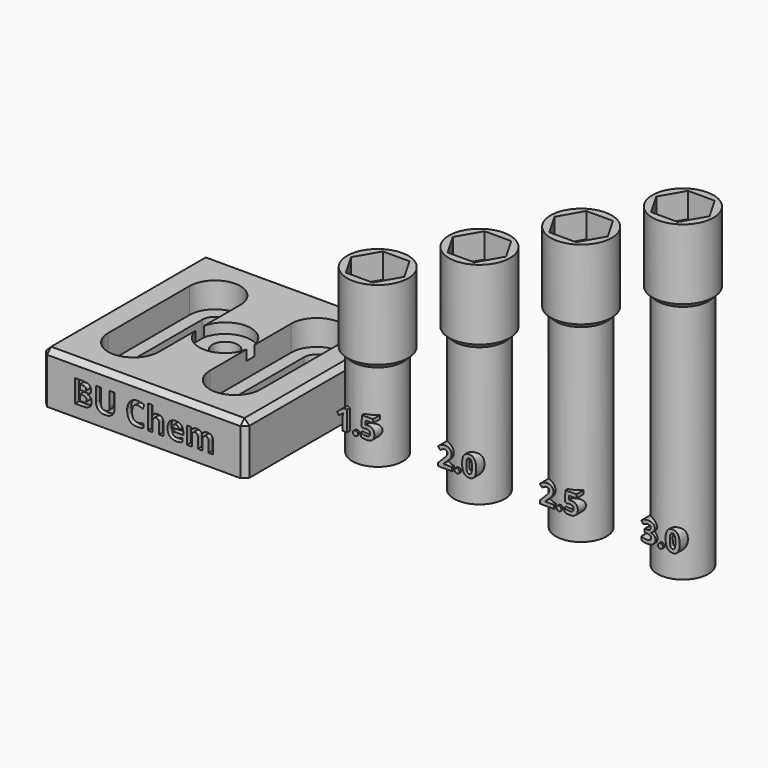
from build123d import *

# Parameters (mm, degrees)
F0_W          = 50.8
F0_H          = 50.8
F0_R          = 3.175
F1_DEPTH      = 12.7
F3_DEPTH      = 6.35
F2_R          = 3.175
F4_DEPTH      = 2.54
F5_SIZE       = 1.27
F6_DEPTH      = 5.08
F7_TEXT_SIZE  = 7.8593141451
F8_DEPTH      = 1.27
F0_R_2        = 6.35
F0_R_3        = 3.429
F9_DEPTH      = 47.244
F10_DEPTH     = 21.844
F11_DEPTH     = 34.544
F12_DEPTH     = 59.944
F13_R         = 7.62
F13_R_2       = 6.35
F13_R_3       = 3.429
F14_DEPTH     = 18.796
F15_R         = 7.62
F15_R_2       = 6.35
F15_R_3       = 3.429
F16_DEPTH     = 18.796
F17_R         = 7.62
F17_R_2       = 6.35
F17_R_3       = 3.429
F18_DEPTH     = 18.796
F19_R         = 7.62
F19_R_2       = 6.35
F19_R_3       = 3.429
F20_DEPTH     = 18.796
F21_SIZE      = 1.26999
F21_2_SIZE    = 1.26999
F21_3_SIZE    = 1.26999
F21_4_SIZE    = 1.26999
F22_R         = 3.429
F23_DEPTH     = 6.223
F24_R         = 3.429
F25_DEPTH     = 6.223
F26_R         = 3.429
F27_DEPTH     = 6.223
F28_R         = 3.429
F29_DEPTH     = 6.223
F31_TEXT_SIZE = 7.0555555556
F32_DEPTH     = 3.175
F33_DEPTH     = 3.175
F34_DEPTH     = 3.175
F35_DEPTH     = 3.175


# Not quite as in the source:
# - a fillet or chamfer is up to 0.001 mm smaller than in the source, because OpenCascade refuses the exact size
# - Text() gives the source's letters only with a copy of the font that has no kerning and outlines rounded to 1/6400 em; it was checked with that copy


with BuildPart() as f1:
    # F0 (on Top) → F1 (new body)
    with BuildSketch(Plane.XY):
        Rectangle(F0_W, F0_H)
        with BuildLine():
            Line((-9.525, 12.7), (-9.525, -12.7))
            ThreePointArc((-9.525, -12.7), (-12.7, -15.875), (-15.875, -12.7))
            Line((-15.875, -12.7), (-15.875, 12.7))
            ThreePointArc((-15.875, 12.7), (-12.7, 15.875), (-9.525, 12.7))
        make_face(mode=Mode.SUBTRACT)
        Polygon((0, 6.604), (5.7192317666, 3.302), (5.7192317666, -3.302), (0, -6.604), (-5.7192317666, -3.302), (-5.7192317666, 3.302), align=None, mode=Mode.SUBTRACT)
        with BuildLine():
            Line((15.875, 12.7), (15.875, -12.7))
            ThreePointArc((15.875, -12.7), (12.7, -15.875), (9.525, -12.7))
            Line((9.525, -12.7), (9.525, 12.7))
            ThreePointArc((9.525, 12.7), (12.7, 15.875), (15.875, 12.7))
        make_face(mode=Mode.SUBTRACT)
        Polygon((5.7192317666, -3.302), (5.7192317666, 3.302), (0, 6.604), (-5.7192317666, 3.302), (-5.7192317666, -3.302), (0, -6.604), align=None)
        Circle(F0_R, mode=Mode.SUBTRACT)
    extrude(amount=F1_DEPTH)

    # F2 (on face) → F3 (cut)
    with BuildSketch(Plane.XY.offset(12.7)):
        with BuildLine():
            ThreePointArc((-9.525, 7.200738686), (-7.200738686, 9.525), (-6.35, 12.7))
            ThreePointArc((-6.35, 12.7), (-12.7, 19.05), (-19.05, 12.7))
            ThreePointArc((-19.05, 12.7), (-18.199261314, 9.525), (-15.875, 7.200738686))
            Line((-15.875, 7.200738686), (-15.875, 12.7))
            ThreePointArc((-15.875, 12.7), (-12.7, 15.875), (-9.525, 12.7))
            Line((-9.525, 12.7), (-9.525, 7.200738686))
        make_face()
        with BuildLine():
            Line((-6.35, 1.2763342039), (-6.35, 12.7))
            ThreePointArc((-6.35, 12.7), (-7.200738686, 9.525), (-9.525, 7.200738686))
            Line((-9.525, 7.200738686), (-9.525, -7.200738686))
            ThreePointArc((-9.525, -7.200738686), (-7.200738686, -9.525), (-6.35, -12.7))
            Line((-6.35, -12.7), (-6.35, -1.2763342039))
            ThreePointArc((-6.35, -1.2763342039), (-6.477, 0), (-6.35, 1.2763342039))
        make_face()
        with BuildLine():
            ThreePointArc((-15.875, 7.200738686), (-18.199261314, 9.525), (-19.05, 12.7))
            Line((-19.05, 12.7), (-19.05, -12.7))
            ThreePointArc((-19.05, -12.7), (-18.199261314, -9.525), (-15.875, -7.200738686))
            Line((-15.875, -7.200738686), (-15.875, 7.200738686))
        make_face()
        with BuildLine():
            ThreePointArc((-15.875, 7.200738686), (-12.7, 6.35), (-9.525, 7.200738686))
            Line((-9.525, 7.200738686), (-9.525, 12.7))
            ThreePointArc((-9.525, 12.7), (-12.7, 15.875), (-15.875, 12.7))
            Line((-15.875, 12.7), (-15.875, 7.200738686))
        make_face()
        with BuildLine():
            Line((-6.35, -1.2763342039), (-6.35, 1.2763342039))
            ThreePointArc((-6.35, 1.2763342039), (-6.477, 0), (-6.35, -1.2763342039))
        make_face()
        with BuildLine():
            ThreePointArc((-15.875, -7.200738686), (-18.199261314, -9.525), (-19.05, -12.7))
            ThreePointArc((-19.05, -12.7), (-12.7, -19.05), (-6.35, -12.7))
            ThreePointArc((-6.35, -12.7), (-7.200738686, -9.525), (-9.525, -7.200738686))
            Line((-9.525, -7.200738686), (-9.525, -12.7))
            ThreePointArc((-9.525, -12.7), (-12.7, -15.875), (-15.875, -12.7))
            Line((-15.875, -12.7), (-15.875, -7.200738686))
        make_face()
        with BuildLine():
            Line((-9.525, -12.7), (-9.525, -7.200738686))
            ThreePointArc((-9.525, -7.200738686), (-12.7, -6.35), (-15.875, -7.200738686))
            Line((-15.875, -7.200738686), (-15.875, -12.7))
            ThreePointArc((-15.875, -12.7), (-12.7, -15.875), (-9.525, -12.7))
        make_face()
        with BuildLine():
            Line((6.35, 12.7), (6.35, 1.2763342039))
            ThreePointArc((6.35, 1.2763342039), (6.4451717976, 0.6413185636), (6.477, 0))
            ThreePointArc((6.477, 0), (6.4451717976, -0.6413185636), (6.35, -1.2763342039))
            Line((6.35, -1.2763342039), (6.35, -12.7))
            ThreePointArc((6.35, -12.7), (7.200738686, -9.525), (9.525, -7.200738686))
            Line((9.525, -7.200738686), (9.525, 7.200738686))
            ThreePointArc((9.525, 7.200738686), (7.200738686, 9.525), (6.35, 12.7))
        make_face()
        with BuildLine():
            ThreePointArc((6.477, 0), (6.4451717976, 0.6413185636), (6.35, 1.2763342039))
            Line((6.35, 1.2763342039), (6.35, -1.2763342039))
            ThreePointArc((6.35, -1.2763342039), (6.4451717976, -0.6413185636), (6.477, 0))
        make_face()
        with BuildLine():
            ThreePointArc((19.05, 12.7), (12.7, 19.05), (6.35, 12.7))
            ThreePointArc((6.35, 12.7), (7.200738686, 9.525), (9.525, 7.200738686))
            Line((9.525, 7.200738686), (9.525, 12.7))
            ThreePointArc((9.525, 12.7), (12.7, 15.875), (15.875, 12.7))
            Line((15.875, 12.7), (15.875, 7.200738686))
            ThreePointArc((15.875, 7.200738686), (18.199261314, 9.525), (19.05, 12.7))
        make_face()
        with BuildLine():
            Line((19.05, -12.7), (19.05, 12.7))
            ThreePointArc((19.05, 12.7), (18.199261314, 9.525), (15.875, 7.200738686))
            Line((15.875, 7.200738686), (15.875, -7.200738686))
            ThreePointArc((15.875, -7.200738686), (18.199261314, -9.525), (19.05, -12.7))
        make_face()
        with BuildLine():
            Line((9.525, 12.7), (9.525, 7.200738686))
            ThreePointArc((9.525, 7.200738686), (12.7, 6.35), (15.875, 7.200738686))
            Line((15.875, 7.200738686), (15.875, 12.7))
            ThreePointArc((15.875, 12.7), (12.7, 15.875), (9.525, 12.7))
        make_face()
        with BuildLine():
            ThreePointArc((9.525, -7.200738686), (7.200738686, -9.525), (6.35, -12.7))
            ThreePointArc((6.35, -12.7), (12.7, -19.05), (19.05, -12.7))
            ThreePointArc((19.05, -12.7), (18.199261314, -9.525), (15.875, -7.200738686))
            Line((15.875, -7.200738686), (15.875, -12.7))
            ThreePointArc((15.875, -12.7), (12.7, -15.875), (9.525, -12.7))
            Line((9.525, -12.7), (9.525, -7.200738686))
        make_face()
        with BuildLine():
            ThreePointArc((15.875, -7.200738686), (12.7, -6.35), (9.525, -7.200738686))
            Line((9.525, -7.200738686), (9.525, -12.7))
            ThreePointArc((9.525, -12.7), (12.7, -15.875), (15.875, -12.7))
            Line((15.875, -12.7), (15.875, -7.200738686))
        make_face()
    extrude(amount=-F3_DEPTH, mode=Mode.SUBTRACT)

    # F2 (on face) → F4 (cut)
    with BuildSketch(Plane.XY.offset(12.7)):
        with BuildLine():
            Line((-6.35, -1.2763342039), (-6.35, 1.2763342039))
            ThreePointArc((-6.35, 1.2763342039), (-6.477, 0), (-6.35, -1.2763342039))
        make_face()
        with BuildLine():
            ThreePointArc((6.35, 1.2763342039), (0, 6.477), (-6.35, 1.2763342039))
            Line((-6.35, 1.2763342039), (-6.35, -1.2763342039))
            ThreePointArc((-6.35, -1.2763342039), (0, -6.477), (6.35, -1.2763342039))
            Line((6.35, -1.2763342039), (6.35, 1.2763342039))
        make_face()
        Circle(F2_R, mode=Mode.SUBTRACT)
        with BuildLine():
            ThreePointArc((6.477, 0), (6.4451717976, 0.6413185636), (6.35, 1.2763342039))
            Line((6.35, 1.2763342039), (6.35, -1.2763342039))
            ThreePointArc((6.35, -1.2763342039), (6.4451717976, -0.6413185636), (6.477, 0))
        make_face()
    extrude(amount=-F4_DEPTH, mode=Mode.SUBTRACT)

    # F5
    f5_edges = [f1.edges().sort_by_distance(p)[0] for p in [
        (0, -25.4, 12.7),
        (-25.4, 0, 12.7),
        (0, 25.4, 12.7),
        (25.4, 0, 12.7),
        (-25.4, -25.4, 6.35),
        (25.4, -25.4, 6.35),
        (-25.4, 25.4, 6.35),
        (25.4, 25.4, 6.35),
    ]]
    chamfer(f5_edges, length=F5_SIZE)

    # F0 (on Top) → F6 (cut)
    with BuildSketch(Plane.XY):
        Polygon((5.7192317666, -3.302), (5.7192317666, 3.302), (0, 6.604), (-5.7192317666, 3.302), (-5.7192317666, -3.302), (0, -6.604), align=None)
        Circle(F0_R, mode=Mode.SUBTRACT)
    extrude(amount=F6_DEPTH, mode=Mode.SUBTRACT)

    # F7 (on face) → F8 (cut)
    with BuildSketch(Plane.XZ.offset(25.4)):
        with Locations((-17.8596773858, 2.9821679927)):
            Text('BU Chem', F7_TEXT_SIZE, font='Open Sans', font_style=FontStyle.BOLD, text_align=(TextAlign.LEFT, TextAlign.BOTTOM))
    extrude(amount=-F8_DEPTH, mode=Mode.SUBTRACT)


with BuildPart() as f9:
    # F0 (on Top) → F9 (new body)
    with BuildSketch(Plane.XY):
        with Locations((88.9, 0)):
            Circle(F0_R_2)
        with Locations((88.9, 0)):
            Circle(F0_R_3, mode=Mode.SUBTRACT)
    extrude(amount=F9_DEPTH)

    # F17 (on face) → F18 (join)
    with BuildSketch(Plane.XY.offset(47.244)):
        with Locations((88.9, 0)):
            Circle(F17_R)
        with Locations((88.9, 0)):
            Circle(F17_R_2, mode=Mode.SUBTRACT)
        with Locations((88.9, 0)):
            Circle(F17_R_2)
        with Locations((88.9, 0)):
            Circle(F17_R_3, mode=Mode.SUBTRACT)
    extrude(amount=F18_DEPTH)

    # F21 (size 1.27 in the source; OpenCascade refuses exactly that, so slightly less here)
    f21_edges = [f9.edges().sort_by_distance(p)[0] for p in [
        (81.28, 0, 47.244),
    ]]
    chamfer(f21_edges, length=F21_SIZE)

    # F26 (on face) → F27 (cut)
    with BuildSketch(Plane.XY.offset(66.04)):
        Polygon((92.2274, -5.7632258571), (95.5548, 0), (92.2274, 5.7632258571), (85.5726, 5.7632258571), (82.2452, 0), (85.5726, -5.7632258571), align=None)
        with Locations((88.9, 0)):
            Circle(F26_R, mode=Mode.SUBTRACT)
    extrude(amount=-F27_DEPTH, mode=Mode.SUBTRACT)

    # F31 (on offset) → F34 (join)
    with BuildSketch(Plane.XZ.offset(6.858)):
        with Locations((83.7962977431, 6.35)):
            Text('2.5', F31_TEXT_SIZE, font='Open Sans', font_style=FontStyle.BOLD, text_align=(TextAlign.LEFT, TextAlign.BOTTOM))
    extrude(amount=-F34_DEPTH)


with BuildPart() as f10:
    # F0 (on Top) → F10 (new body)
    with BuildSketch(Plane.XY):
        with Locations((38.1, 0)):
            Circle(F0_R_2)
        with Locations((38.1, 0)):
            Circle(F0_R_3, mode=Mode.SUBTRACT)
    extrude(amount=F10_DEPTH)

    # F13 (on face) → F14 (join)
    with BuildSketch(Plane.XY.offset(21.844)):
        with Locations((38.1, 0)):
            Circle(F13_R)
        with Locations((38.1, 0)):
            Circle(F13_R_2, mode=Mode.SUBTRACT)
        with Locations((38.1, 0)):
            Circle(F13_R_2)
        with Locations((38.1, 0)):
            Circle(F13_R_3, mode=Mode.SUBTRACT)
    extrude(amount=F14_DEPTH)

    # F21#2 (size 1.27 in the source; OpenCascade refuses exactly that, so slightly less here)
    f21_2_edges = [f10.edges().sort_by_distance(p)[0] for p in [
        (30.48, 0, 21.844),
    ]]
    chamfer(f21_2_edges, length=F21_2_SIZE)

    # F22 (on face) → F23 (cut)
    with BuildSketch(Plane.XY.offset(40.64)):
        Polygon((41.4274, -5.7632258571), (44.7548, 0), (41.4274, 5.7632258571), (34.7726, 5.7632258571), (31.4452, 0), (34.7726, -5.7632258571), align=None)
        with Locations((38.1, 0)):
            Circle(F22_R, mode=Mode.SUBTRACT)
    extrude(amount=-F23_DEPTH, mode=Mode.SUBTRACT)

    # F31 (on offset) → F32 (join)
    with BuildSketch(Plane.XZ.offset(6.858)):
        with Locations((32.9962977431, 6.35)):
            Text('1.5', F31_TEXT_SIZE, font='Open Sans', font_style=FontStyle.BOLD, text_align=(TextAlign.LEFT, TextAlign.BOTTOM))
    extrude(amount=-F32_DEPTH)


with BuildPart() as f11:
    # F0 (on Top) → F11 (new body)
    with BuildSketch(Plane.XY):
        with Locations((63.5, 0)):
            Circle(F0_R_2)
        with Locations((63.5, 0)):
            Circle(F0_R_3, mode=Mode.SUBTRACT)
    extrude(amount=F11_DEPTH)

    # F15 (on face) → F16 (join)
    with BuildSketch(Plane.XY.offset(34.544)):
        with Locations((63.5, 0)):
            Circle(F15_R)
        with Locations((63.5, 0)):
            Circle(F15_R_2, mode=Mode.SUBTRACT)
        with Locations((63.5, 0)):
            Circle(F15_R_2)
        with Locations((63.5, 0)):
            Circle(F15_R_3, mode=Mode.SUBTRACT)
    extrude(amount=F16_DEPTH)

    # F21#3 (size 1.27 in the source; OpenCascade refuses exactly that, so slightly less here)
    f21_3_edges = [f11.edges().sort_by_distance(p)[0] for p in [
        (55.88, 0, 34.544),
    ]]
    chamfer(f21_3_edges, length=F21_3_SIZE)

    # F24 (on face) → F25 (cut)
    with BuildSketch(Plane.XY.offset(53.34)):
        Polygon((66.8274, -5.7632258571), (70.1548, 0), (66.8274, 5.7632258571), (60.1726, 5.7632258571), (56.8452, 0), (60.1726, -5.7632258571), align=None)
        with Locations((63.5, 0)):
            Circle(F24_R, mode=Mode.SUBTRACT)
    extrude(amount=-F25_DEPTH, mode=Mode.SUBTRACT)

    # F31 (on offset) → F33 (join)
    with BuildSketch(Plane.XZ.offset(6.858)):
        with Locations((58.3637760417, 6.35)):
            Text('2.0', F31_TEXT_SIZE, font='Open Sans', font_style=FontStyle.BOLD, text_align=(TextAlign.LEFT, TextAlign.BOTTOM))
    extrude(amount=-F33_DEPTH)


with BuildPart() as f12:
    # F0 (on Top) → F12 (new body)
    with BuildSketch(Plane.XY):
        with Locations((114.3, 0)):
            Circle(F0_R_2)
        with Locations((114.3, 0)):
            Circle(F0_R_3, mode=Mode.SUBTRACT)
    extrude(amount=F12_DEPTH)

    # F19 (on face) → F20 (join)
    with BuildSketch(Plane.XY.offset(59.944)):
        with Locations((114.3, 0)):
            Circle(F19_R)
        with Locations((114.3, 0)):
            Circle(F19_R_2, mode=Mode.SUBTRACT)
        with Locations((114.3, 0)):
            Circle(F19_R_2)
        with Locations((114.3, 0)):
            Circle(F19_R_3, mode=Mode.SUBTRACT)
    extrude(amount=F20_DEPTH)

    # F21#4 (size 1.27 in the source; OpenCascade refuses exactly that, so slightly less here)
    f21_4_edges = [f12.edges().sort_by_distance(p)[0] for p in [
        (106.68, 0, 59.944),
    ]]
    chamfer(f21_4_edges, length=F21_4_SIZE)

    # F28 (on face) → F29 (cut)
    with BuildSketch(Plane.XY.offset(78.74)):
        Polygon((117.6274, -5.7632258571), (120.9548, 0), (117.6274, 5.7632258571), (110.9726, 5.7632258571), (107.6452, 0), (110.9726, -5.7632258571), align=None)
        with Locations((114.3, 0)):
            Circle(F28_R, mode=Mode.SUBTRACT)
    extrude(amount=-F29_DEPTH, mode=Mode.SUBTRACT)

    # F31 (on offset) → F35 (join)
    with BuildSketch(Plane.XZ.offset(6.858)):
        with Locations((109.1637760417, 6.35)):
            Text('3.0', F31_TEXT_SIZE, font='Open Sans', font_style=FontStyle.BOLD, text_align=(TextAlign.LEFT, TextAlign.BOTTOM))
    extrude(amount=-F35_DEPTH)


solid = Compound([f1.part, f9.part, f10.part, f11.part, f12.part])
